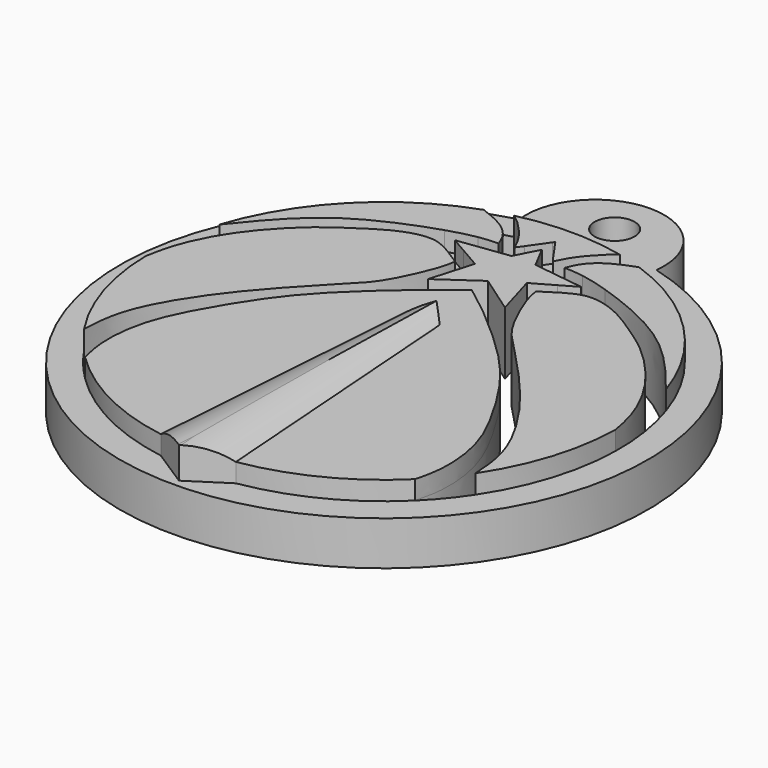
from build123d import *

# Parameters (mm, degrees)
F0_R        = 1.5875
F1_DEPTH    = 3.5
F2_DEPTH    = 5
F3_DEPTH    = 5
F4_DEPTH    = 6
F5_T1_DEPTH = 37.3647576307
F5_T3_DEPTH = 37.3647576307


# Not quite as in the source:
# - a fillet or chamfer that OpenCascade refuses, or shapes differently, is made with other operations: its cross-section is extruded or revolved along the edge and cut away or added


with BuildPart() as f1:
    # F0 (on Top) → F1 (new body)
    with BuildSketch(Plane.XY):
        with BuildLine():
            ThreePointArc((-10.6217474034, 18.1667311499), (-17.945936649, -18.7789449236), (15.8308902232, -2.1130307549))
            ThreePointArc((15.8308902232, -2.1130307549), (11.4968043919, 10.6637961173), (0.2835278497, 18.1667311499))
            ThreePointArc((0.2835278497, 18.1667311499), (-5.1691097768, 18.8869692451), (-10.6217474034, 18.1667311499))
        make_face()
        with BuildLine():
            ThreePointArc((7.9582883799, -15.4297572305), (3.287871388, -18.7906581631), (-2.183307789, -20.5724124585))
            Line((-2.183307789, -20.5724124585), (-5.1691097768, -22.5024949759))
            Line((-5.1691097768, -22.5024949759), (-8.1549117647, -20.5724124585))
            ThreePointArc((-8.1549117647, -20.5724124585), (-13.6260909417, -18.7906581631), (-18.2965079335, -15.4297572305))
            ThreePointArc((-18.2965079335, -15.4297572305), (-19.5901108284, -14.0167492942), (-20.7323538336, -12.4788023528))
            ThreePointArc((-20.7323538336, -12.4788023528), (-23.0163230381, -7.6934218882), (-23.8652020884, -2.4593235058))
            ThreePointArc((-23.8652020884, -2.4593235058), (-23.6597566898, 0.672604385), (-22.9333688875, 3.7260517623))
            ThreePointArc((-22.9333688875, 3.7260517623), (-18.5175516222, 10.9821166934), (-11.3474056156, 15.5361178626))
            ThreePointArc((-11.3474056156, 15.5361178626), (-10.3705266124, 15.8482901681), (-9.3780024098, 16.1064371078))
            ThreePointArc((-9.3780024098, 16.1064371078), (-5.1691097768, 16.5862683334), (-0.9602171439, 16.1064371078))
            ThreePointArc((-0.9602171439, 16.1064371078), (0.0323070587, 15.8482901681), (1.0091860619, 15.5361178626))
            ThreePointArc((1.0091860619, 15.5361178626), (8.1793320686, 10.9821166934), (12.5951493338, 3.7260517623))
            ThreePointArc((12.5951493338, 3.7260517623), (13.3215371361, 0.672604385), (13.5269825347, -2.4593235058))
            ThreePointArc((13.5269825347, -2.4593235058), (12.6781034844, -7.6934218882), (10.3941342799, -12.4788023528))
            ThreePointArc((10.3941342799, -12.4788023528), (9.2518912747, -14.0167492942), (7.9582883799, -15.4297572305))
        make_face(mode=Mode.SUBTRACT)
        with BuildLine():
            ThreePointArc((-10.6217474034, 18.1667311499), (-5.1691097768, 18.8869692451), (0.2835278497, 18.1667311499))
            ThreePointArc((0.2835278497, 18.1667311499), (-5.1691097768, 24.3869692451), (-10.6217474034, 18.1667311499))
        make_face()
        with Locations((-5.1691097768, 20.8305809647)):
            Circle(F0_R, mode=Mode.SUBTRACT)
        with BuildLine():
            Line((-3.8073558551, 1.7333009746), (-2.183307789, -20.5724124585))
            ThreePointArc((-2.183307789, -20.5724124585), (3.287871388, -18.7906581631), (7.9582883799, -15.4297572305))
            add(Edge.make_bspline(
                [(7.9582883799, -15.4297572305), (8.1268709506, -14.7676605332), (8.5082883638, -13.2407756078), (8.2126910715, -9.4168255285), (6.2922035042, -5.5331151551), (3.6366838506, -1.3148563239), (0.7165543738, 1.7563956632), (-2.917726549, 4.9627751379), (-4.4908734673, 6.1293824819), (-5.1691097768, 6.6323461942)],
                knots=[0, 0, 0, 0, 0.1082288162, 0.2489656613, 0.4027377179, 0.5651921966, 0.718242587, 0.878508978, 1, 1, 1, 1], degree=3))
            add(Edge.make_bspline(
                [(-18.2965079335, -15.4297572305), (-18.4650905043, -14.7676605332), (-18.8465079175, -13.2407756078), (-18.5509106252, -9.4168255285), (-16.6304230579, -5.5331151551), (-13.9749034043, -1.3148563239), (-11.0547739275, 1.7563956632), (-7.4204930047, 4.9627751379), (-5.8473460864, 6.1293824819), (-5.1691097768, 6.6323461942)],
                knots=[0, 0, 0, 0, 0.1082288162, 0.2489656613, 0.4027377179, 0.5651921966, 0.718242587, 0.878508978, 1, 1, 1, 1], degree=3))
            ThreePointArc((-18.2965079335, -15.4297572305), (-13.6260909417, -18.7906581631), (-8.1549117647, -20.5724124585))
            Line((-8.1549117647, -20.5724124585), (-6.5308636986, 1.7333009746))
            Line((-6.5308636986, 1.7333009746), (-5.1691097768, 3.1168696005))
            Line((-5.1691097768, 3.1168696005), (-3.8073558551, 1.7333009746))
        make_face()
    extrude(amount=F1_DEPTH)



with BuildPart() as f1b:
    # F0 (on Top) → F1, piece 2 (new body)
    with BuildSketch(Plane.XY):
        with BuildLine():
            add(Edge.make_bspline(
                [(-0.6594804695, 9.8146022568), (-0.3132768964, 10.0157483029), (0.352786766, 10.3622623091), (0.9138670644, 10.4710599705), (1.1655195088, 10.4825454153)],
                knots=[0.1007074481, 0.1007074481, 0.1007074481, 0.1007074481, 0.167295478, 0.2177868881, 0.2177868881, 0.2177868881, 0.2177868881], degree=3))
            ThreePointArc((1.1655195088, 10.4825454153), (1.3107635614, 10.8394988108), (1.3602674152, 11.2216779962))
            ThreePointArc((1.3602674152, 11.2216779962), (1.3218671337, 11.558911243), (1.2086323982, 11.878878021))
            add(Edge.make_bspline(
                [(1.2086323982, 11.878878021), (0.6116951762, 12.0699599932), (-0.1950310099, 12.2945209177), (-0.8204575004, 12.4165577745), (-1.0045308117, 12.4472896912)],
                knots=[0.7363290583, 0.7363290583, 0.7363290583, 0.7363290583, 0.8238242503, 0.864376936, 0.864376936, 0.864376936, 0.864376936], degree=3))
            ThreePointArc((-1.0045308117, 12.4472896912), (-1.4231996557, 11.9980234592), (-1.626745872, 11.4186335336))
            Line((-1.626745872, 11.4186335336), (-0.1397325848, 11.2216779962))
            Line((-0.1397325848, 11.2216779962), (-1.441368461, 10.4761955713))
            ThreePointArc((-1.441368461, 10.4761955713), (-1.1086423482, 10.076595523), (-0.6594804695, 9.8146022568))
        make_face()
    extrude(amount=F1_DEPTH)


with BuildPart() as f1c:
    # F0 (on Top) → F1, piece 3 (new body)
    with BuildSketch(Plane.XY):
        with BuildLine():
            ThreePointArc((-11.5468519519, 11.878878021), (-11.6977724933, 11.1753863528), (-11.5037390625, 10.4825454153))
            add(Edge.make_bspline(
                [(-9.6787390842, 9.8146022568), (-10.0249426572, 10.0157483029), (-10.6910063197, 10.3622623091), (-11.2520866181, 10.4710599705), (-11.5037390625, 10.4825454153)],
                knots=[0.1007074481, 0.1007074481, 0.1007074481, 0.1007074481, 0.167295478, 0.2177868881, 0.2177868881, 0.2177868881, 0.2177868881], degree=3))
            ThreePointArc((-9.6787390842, 9.8146022568), (-9.2295772055, 10.076595523), (-8.8968510927, 10.4761955713))
            Line((-8.8968510927, 10.4761955713), (-10.1984869689, 11.2216779962))
            Line((-10.1984869689, 11.2216779962), (-8.7114736817, 11.4186335336))
            ThreePointArc((-8.7114736817, 11.4186335336), (-8.915019898, 11.9980234592), (-9.333688742, 12.4472896912))
            add(Edge.make_bspline(
                [(-11.5468519519, 11.878878021), (-10.9499147299, 12.0699599932), (-10.1431885437, 12.2945209177), (-9.5177620533, 12.4165577745), (-9.333688742, 12.4472896912)],
                knots=[0.7363290583, 0.7363290583, 0.7363290583, 0.7363290583, 0.8238242503, 0.864376936, 0.864376936, 0.864376936, 0.864376936], degree=3))
        make_face()
    extrude(amount=F1_DEPTH)


with BuildPart() as f1d:
    # F0 (on Top) → F1, piece 4 (new body)
    with BuildSketch(Plane.XY):
        with BuildLine():
            ThreePointArc((-4.6168923991, 12.5363375369), (-4.2373473906, 12.8481972521), (-4.0154397933, 13.2864527868))
            add(Edge.make_bspline(
                [(-4.0154397933, 13.2864527868), (-4.1692049041, 13.4990699244), (-4.5365971578, 14.0110964025), (-4.8706595062, 14.4992054582), (-5.0654287777, 14.7850824568)],
                knots=[0.2267202191, 0.2267202191, 0.2267202191, 0.2267202191, 0.5150033084, 0.9268445188, 0.9268445188, 0.9268445188, 0.9268445188], degree=3))
            ThreePointArc((-5.0654287777, 14.7850824568), (-5.1691097768, 14.7895914288), (-5.272790776, 14.7850824568))
            add(Edge.make_bspline(
                [(-6.3227797603, 13.2864527868), (-6.1690146496, 13.4990699244), (-5.8016223959, 14.0110964025), (-5.4675600475, 14.4992054582), (-5.272790776, 14.7850824568)],
                knots=[0.2267202191, 0.2267202191, 0.2267202191, 0.2267202191, 0.5150033084, 0.9268445188, 0.9268445188, 0.9268445188, 0.9268445188], degree=3))
            ThreePointArc((-6.3227797603, 13.2864527868), (-6.1008721631, 12.8481972521), (-5.7213271546, 12.5363375369))
            Line((-5.7213271546, 12.5363375369), (-5.2771929481, 13.3880313451))
            Line((-5.2771929481, 13.3880313451), (-5.1691097768, 13.5952970013))
            Line((-5.1691097768, 13.5952970013), (-4.6168923991, 12.5363375369))
        make_face()
        with BuildLine():
            ThreePointArc((-5.7213271546, 12.5363375369), (-5.1691097768, 12.4010025738), (-4.6168923991, 12.5363375369))
            Line((-4.6168923991, 12.5363375369), (-5.1691097768, 13.5952970013))
            Line((-5.1691097768, 13.5952970013), (-5.2771929481, 13.3880313451))
            Line((-5.2771929481, 13.3880313451), (-5.7213271546, 12.5363375369))
        make_face()
    extrude(amount=F1_DEPTH)


with BuildPart() as f1_1:
    add(f1.part)

    add(f1b.part)  # F2 merges F1b

    add(f1c.part)  # F2 merges F1c

    add(f1d.part)  # F2 merges F1d
    # F0 (on Top) → F2 (join)
    with BuildSketch(Plane.XY):
        with BuildLine():
            Line((-3.8073558551, 1.7333009746), (-2.183307789, -20.5724124585))
            ThreePointArc((-2.183307789, -20.5724124585), (3.287871388, -18.7906581631), (7.9582883799, -15.4297572305))
            add(Edge.make_bspline(
                [(7.9582883799, -15.4297572305), (8.1268709506, -14.7676605332), (8.5082883638, -13.2407756078), (8.2126910715, -9.4168255285), (6.2922035042, -5.5331151551), (3.6366838506, -1.3148563239), (0.7165543738, 1.7563956632), (-2.917726549, 4.9627751379), (-4.4908734673, 6.1293824819), (-5.1691097768, 6.6323461942)],
                knots=[0, 0, 0, 0, 0.1082288162, 0.2489656613, 0.4027377179, 0.5651921966, 0.718242587, 0.878508978, 1, 1, 1, 1], degree=3))
            add(Edge.make_bspline(
                [(-18.2965079335, -15.4297572305), (-18.4650905043, -14.7676605332), (-18.8465079175, -13.2407756078), (-18.5509106252, -9.4168255285), (-16.6304230579, -5.5331151551), (-13.9749034043, -1.3148563239), (-11.0547739275, 1.7563956632), (-7.4204930047, 4.9627751379), (-5.8473460864, 6.1293824819), (-5.1691097768, 6.6323461942)],
                knots=[0, 0, 0, 0, 0.1082288162, 0.2489656613, 0.4027377179, 0.5651921966, 0.718242587, 0.878508978, 1, 1, 1, 1], degree=3))
            ThreePointArc((-18.2965079335, -15.4297572305), (-13.6260909417, -18.7906581631), (-8.1549117647, -20.5724124585))
            Line((-8.1549117647, -20.5724124585), (-6.5308636986, 1.7333009746))
            Line((-6.5308636986, 1.7333009746), (-5.1691097768, 3.1168696005))
            Line((-5.1691097768, 3.1168696005), (-3.8073558551, 1.7333009746))
        make_face()
        with BuildLine():
            add(Edge.make_bspline(
                [(10.3941342799, -12.4788023528), (10.3452942412, -11.6564178564), (10.2266128746, -9.932430264), (9.1917748323, -7.0399501633), (6.2457162099, -2.4988215533), (1.6434245686, 2.3032416473), (-0.1345824017, 4.0356531353), (-1.7597757021, 7.7058988796), (-1.8958501186, 8.6475784808), (-1.9455046584, 8.991218172)],
                knots=[0, 0, 0, 0, 0.1218601492, 0.2546294874, 0.4377987849, 0.6359398562, 0.762473885, 0.9132895155, 1, 1, 1, 1], degree=3))
            ThreePointArc((10.3941342799, -12.4788023528), (12.6781034844, -7.6934218882), (13.5269825347, -2.4593235058))
            add(Edge.make_bspline(
                [(1.1655195088, 10.4825454153), (1.3095245657, 10.4891178217), (1.9782324137, 10.4662598398), (3.6604034661, 10.0126361433), (6.3600557238, 8.1858017478), (8.468040147, 6.6827991764), (11.432590494, 3.4209544025), (13.0749001344, -0.038175844), (13.3944902979, -1.7190671567), (13.5269825347, -2.4593235058)],
                knots=[0.2177868881, 0.2177868881, 0.2177868881, 0.2177868881, 0.2466799847, 0.3490657461, 0.4784660181, 0.5963471121, 0.7469989964, 0.8886972052, 1, 1, 1, 1], degree=3))
            ThreePointArc((1.1655195088, 10.4825454153), (0.3758168612, 9.8130585413), (-0.6594804695, 9.8146022568))
            add(Edge.make_bspline(
                [(-1.9455046584, 8.991218172), (-1.6687696745, 9.1788138573), (-1.2974280921, 9.4305422257), (-0.7928309739, 9.737124932), (-0.6594804695, 9.8146022568)],
                knots=[0, 0, 0, 0, 0.075059107, 0.1007074481, 0.1007074481, 0.1007074481, 0.1007074481], degree=3))
        make_face()
        with BuildLine():
            add(Edge.make_bspline(
                [(12.5951493338, 3.7260517623), (11.837319685, 4.6792052854), (10.1727952981, 6.7348601777), (6.9410883324, 9.6905588931), (2.79917555, 11.3697388499), (1.2086323982, 11.878878021)],
                knots=[0, 0, 0, 0, 0.2320938274, 0.5031975443, 0.7363290583, 0.7363290583, 0.7363290583, 0.7363290583], degree=3))
            ThreePointArc((12.5951493338, 3.7260517623), (8.1793320686, 10.9821166934), (1.0091860619, 15.5361178626))
            add(Edge.make_bspline(
                [(-2.5381853063, 12.5784734264), (-2.4197419628, 12.891192737), (-2.1668564437, 13.5586539752), (-1.2444477594, 14.5311057124), (0.0078417422, 15.1550512291), (0.6915665814, 15.4186675749), (1.0091860619, 15.5361178626)],
                knots=[0, 0, 0, 0, 0.2315172069, 0.4938081985, 0.7644978013, 1, 1, 1, 1], degree=3))
            add(Edge.make_bspline(
                [(-1.0045308117, 12.4472896912), (-1.620139519, 12.5500684992), (-2.0791736657, 12.5642963988), (-2.5381853063, 12.5784734264)],
                knots=[0.864376936, 0.864376936, 0.864376936, 0.864376936, 1, 1, 1, 1], degree=3))
            ThreePointArc((-1.0045308117, 12.4472896912), (0.2334056719, 12.6745261787), (1.2086323982, 11.878878021))
        make_face()
        with BuildLine():
            ThreePointArc((-0.6594804695, 9.8146022568), (0.3758168612, 9.8130585413), (1.1655195088, 10.4825454153))
            add(Edge.make_bspline(
                [(-0.6594804695, 9.8146022568), (-0.3132768964, 10.0157483029), (0.352786766, 10.3622623091), (0.9138670644, 10.4710599705), (1.1655195088, 10.4825454153)],
                knots=[0.1007074481, 0.1007074481, 0.1007074481, 0.1007074481, 0.167295478, 0.2177868881, 0.2177868881, 0.2177868881, 0.2177868881], degree=3))
        make_face()
        with BuildLine():
            ThreePointArc((-23.8652020884, -2.4593235058), (-23.0163230381, -7.6934218882), (-20.7323538336, -12.4788023528))
            add(Edge.make_bspline(
                [(-20.7323538336, -12.4788023528), (-20.6835137949, -11.6564178564), (-20.5648324283, -9.932430264), (-19.529994386, -7.0399501633), (-16.5839357635, -2.4988215533), (-11.9816441223, 2.3032416473), (-10.2036371519, 4.0356531353), (-8.5784438516, 7.7058988796), (-8.4423694351, 8.6475784808), (-8.3927148953, 8.991218172)],
                knots=[0, 0, 0, 0, 0.1218601492, 0.2546294874, 0.4377987849, 0.6359398562, 0.762473885, 0.9132895155, 1, 1, 1, 1], degree=3))
            add(Edge.make_bspline(
                [(-8.3927148953, 8.991218172), (-8.6694498791, 9.1788138573), (-9.0407914616, 9.4305422257), (-9.5453885798, 9.737124932), (-9.6787390842, 9.8146022568)],
                knots=[0, 0, 0, 0, 0.075059107, 0.1007074481, 0.1007074481, 0.1007074481, 0.1007074481], degree=3))
            ThreePointArc((-9.6787390842, 9.8146022568), (-10.7140364149, 9.8130585413), (-11.5037390625, 10.4825454153))
            add(Edge.make_bspline(
                [(-11.5037390625, 10.4825454153), (-11.6477441193, 10.4891178217), (-12.3164519674, 10.4662598398), (-13.9986230197, 10.0126361433), (-16.6982752775, 8.1858017478), (-18.8062597007, 6.6827991764), (-21.7708100477, 3.4209544025), (-23.413119688, -0.038175844), (-23.7327098516, -1.7190671567), (-23.8652020884, -2.4593235058)],
                knots=[0.2177868881, 0.2177868881, 0.2177868881, 0.2177868881, 0.2466799847, 0.3490657461, 0.4784660181, 0.5963471121, 0.7469989964, 0.8886972052, 1, 1, 1, 1], degree=3))
        make_face()
        with BuildLine():
            add(Edge.make_bspline(
                [(1.2086323982, 11.878878021), (0.6116951762, 12.0699599932), (-0.1950310099, 12.2945209177), (-0.8204575004, 12.4165577745), (-1.0045308117, 12.4472896912)],
                knots=[0.7363290583, 0.7363290583, 0.7363290583, 0.7363290583, 0.8238242503, 0.864376936, 0.864376936, 0.864376936, 0.864376936], degree=3))
            ThreePointArc((1.2086323982, 11.878878021), (0.2334056719, 12.6745261787), (-1.0045308117, 12.4472896912))
        make_face()
        with BuildLine():
            add(Edge.make_bspline(
                [(-0.9602171439, 16.1064371078), (-1.1965800048, 15.9358141969), (-1.7643121989, 15.503844022), (-3.0700995974, 14.0384146087), (-3.4678370488, 13.175622067), (-3.6495767725, 12.7826062962)],
                knots=[0, 0, 0, 0, 0.2782728656, 0.6692240827, 1, 1, 1, 1], degree=3))
            ThreePointArc((-0.9602171439, 16.1064371078), (-5.1691097768, 16.5862683334), (-9.3780024098, 16.1064371078))
            add(Edge.make_bspline(
                [(-9.3780024098, 16.1064371078), (-9.1416395489, 15.9358141969), (-8.5739073548, 15.503844022), (-7.2681199563, 14.0384146087), (-6.8703825049, 13.175622067), (-6.6886427812, 12.7826062962)],
                knots=[0, 0, 0, 0, 0.2782728656, 0.6692240827, 1, 1, 1, 1], degree=3))
            add(Edge.make_bspline(
                [(-6.6886427812, 12.7826062962), (-6.5661755521, 12.9509231737), (-6.4437083229, 13.1192400511), (-6.3227797603, 13.2864527868)],
                knots=[0, 0, 0, 0, 0.2267202191, 0.2267202191, 0.2267202191, 0.2267202191], degree=3))
            ThreePointArc((-6.3227797603, 13.2864527868), (-6.1472230603, 14.2805951732), (-5.272790776, 14.7850824568))
            add(Edge.make_bspline(
                [(-5.272790776, 14.7850824568), (-5.2381938502, 14.8358628761), (-5.2036518135, 14.8866039073), (-5.1691097768, 14.9373449385)],
                knots=[0.9268445188, 0.9268445188, 0.9268445188, 0.9268445188, 1, 1, 1, 1], degree=3))
            add(Edge.make_bspline(
                [(-5.0654287777, 14.7850824568), (-5.1000257034, 14.8358628761), (-5.1345677401, 14.8866039073), (-5.1691097768, 14.9373449385)],
                knots=[0.9268445188, 0.9268445188, 0.9268445188, 0.9268445188, 1, 1, 1, 1], degree=3))
            ThreePointArc((-5.0654287777, 14.7850824568), (-4.2887221295, 14.4023018155), (-3.9748153493, 13.5952970013))
            ThreePointArc((-3.9748153493, 13.5952970013), (-3.9850150146, 13.4395447186), (-4.0154397933, 13.2864527868))
            add(Edge.make_bspline(
                [(-3.6495767725, 12.7826062962), (-3.7720440016, 12.9509231737), (-3.8945112308, 13.1192400511), (-4.0154397933, 13.2864527868)],
                knots=[0, 0, 0, 0, 0.2267202191, 0.2267202191, 0.2267202191, 0.2267202191], degree=3))
        make_face()
        with BuildLine():
            ThreePointArc((-11.3474056156, 15.5361178626), (-18.5175516222, 10.9821166934), (-22.9333688875, 3.7260517623))
            add(Edge.make_bspline(
                [(-22.9333688875, 3.7260517623), (-22.1755392387, 4.6792052854), (-20.5110148518, 6.7348601777), (-17.2793078861, 9.6905588931), (-13.1373951037, 11.3697388499), (-11.5468519519, 11.878878021)],
                knots=[0, 0, 0, 0, 0.2320938274, 0.5031975443, 0.7363290583, 0.7363290583, 0.7363290583, 0.7363290583], degree=3))
            ThreePointArc((-11.5468519519, 11.878878021), (-10.5716252256, 12.6745261787), (-9.333688742, 12.4472896912))
            add(Edge.make_bspline(
                [(-9.333688742, 12.4472896912), (-8.7180800347, 12.5500684992), (-8.2590458879, 12.5642963988), (-7.8000342473, 12.5784734264)],
                knots=[0.864376936, 0.864376936, 0.864376936, 0.864376936, 1, 1, 1, 1], degree=3))
            add(Edge.make_bspline(
                [(-7.8000342473, 12.5784734264), (-7.9184775909, 12.891192737), (-8.17136311, 13.5586539752), (-9.0937717943, 14.5311057124), (-10.3460612959, 15.1550512291), (-11.0297861351, 15.4186675749), (-11.3474056156, 15.5361178626)],
                knots=[0, 0, 0, 0, 0.2315172069, 0.4938081985, 0.7644978013, 1, 1, 1, 1], degree=3))
        make_face()
        with BuildLine():
            add(Edge.make_bspline(
                [(-9.6787390842, 9.8146022568), (-10.0249426572, 10.0157483029), (-10.6910063197, 10.3622623091), (-11.2520866181, 10.4710599705), (-11.5037390625, 10.4825454153)],
                knots=[0.1007074481, 0.1007074481, 0.1007074481, 0.1007074481, 0.167295478, 0.2177868881, 0.2177868881, 0.2177868881, 0.2177868881], degree=3))
            ThreePointArc((-11.5037390625, 10.4825454153), (-10.7140364149, 9.8130585413), (-9.6787390842, 9.8146022568))
        make_face()
        with BuildLine():
            ThreePointArc((-9.333688742, 12.4472896912), (-10.5716252256, 12.6745261787), (-11.5468519519, 11.878878021))
            add(Edge.make_bspline(
                [(-11.5468519519, 11.878878021), (-10.9499147299, 12.0699599932), (-10.1431885437, 12.2945209177), (-9.5177620533, 12.4165577745), (-9.333688742, 12.4472896912)],
                knots=[0.7363290583, 0.7363290583, 0.7363290583, 0.7363290583, 0.8238242503, 0.864376936, 0.864376936, 0.864376936, 0.864376936], degree=3))
        make_face()
        with BuildLine():
            add(Edge.make_bspline(
                [(-4.0154397933, 13.2864527868), (-4.1692049041, 13.4990699244), (-4.5365971578, 14.0110964025), (-4.8706595062, 14.4992054582), (-5.0654287777, 14.7850824568)],
                knots=[0.2267202191, 0.2267202191, 0.2267202191, 0.2267202191, 0.5150033084, 0.9268445188, 0.9268445188, 0.9268445188, 0.9268445188], degree=3))
            ThreePointArc((-4.0154397933, 13.2864527868), (-3.9850150146, 13.4395447186), (-3.9748153493, 13.5952970013))
            ThreePointArc((-3.9748153493, 13.5952970013), (-4.2887221295, 14.4023018155), (-5.0654287777, 14.7850824568))
        make_face()
        with BuildLine():
            ThreePointArc((-5.7213271546, 12.5363375369), (-5.1691097768, 12.4010025738), (-4.6168923991, 12.5363375369))
            Line((-4.6168923991, 12.5363375369), (-5.1691097768, 13.5952970013))
            Line((-5.1691097768, 13.5952970013), (-5.2771929481, 13.3880313451))
            Line((-5.2771929481, 13.3880313451), (-5.7213271546, 12.5363375369))
        make_face()
        with BuildLine():
            ThreePointArc((-5.272790776, 14.7850824568), (-6.1472230603, 14.2805951732), (-6.3227797603, 13.2864527868))
            add(Edge.make_bspline(
                [(-6.3227797603, 13.2864527868), (-6.1690146496, 13.4990699244), (-5.8016223959, 14.0110964025), (-5.4675600475, 14.4992054582), (-5.272790776, 14.7850824568)],
                knots=[0.2267202191, 0.2267202191, 0.2267202191, 0.2267202191, 0.5150033084, 0.9268445188, 0.9268445188, 0.9268445188, 0.9268445188], degree=3))
        make_face()
    extrude(amount=F2_DEPTH)

    # F0 (on Top) → F3 (join)
    with BuildSketch(Plane.XY):
        Polygon((-5.1691097768, -22.5024949759), (-2.183307789, -20.5724124585), (-3.8073558551, 1.7333009746), (-5.1691097768, 3.1168696005), (-6.5308636986, 1.7333009746), (-8.1549117647, -20.5724124585), align=None)
        with BuildLine():
            ThreePointArc((-1.626745872, 11.4186335336), (-1.61153025, 10.9321756081), (-1.441368461, 10.4761955713))
            Line((-1.441368461, 10.4761955713), (-0.1397325848, 11.2216779962))
            Line((-0.1397325848, 11.2216779962), (-1.626745872, 11.4186335336))
        make_face()
        with BuildLine():
            Line((-3.1067568068, 9.52238217), (-1.441368461, 10.4761955713))
            ThreePointArc((-1.441368461, 10.4761955713), (-1.61153025, 10.9321756081), (-1.626745872, 11.4186335336))
            Line((-1.626745872, 11.4186335336), (-4.2126474162, 11.7611372843))
            Line((-4.2126474162, 11.7611372843), (-4.6168923991, 12.5363375369))
            ThreePointArc((-4.6168923991, 12.5363375369), (-5.1691097768, 12.4010025738), (-5.7213271546, 12.5363375369))
            Line((-5.7213271546, 12.5363375369), (-6.1255721375, 11.7611372843))
            Line((-6.1255721375, 11.7611372843), (-8.7114736817, 11.4186335336))
            ThreePointArc((-8.7114736817, 11.4186335336), (-8.7017371683, 11.3203696099), (-8.6984869689, 11.2216779962))
            ThreePointArc((-8.6984869689, 11.2216779962), (-8.7489260329, 10.8359668441), (-8.8968510927, 10.4761955713))
            Line((-8.8968510927, 10.4761955713), (-7.2314627469, 9.52238217))
            Line((-7.2314627469, 9.52238217), (-8.2294614986, 6.0968184844))
            Line((-8.2294614986, 6.0968184844), (-5.1691097768, 8.2276808098))
            Line((-5.1691097768, 8.2276808098), (-2.1087580551, 6.0968184844))
            Line((-2.1087580551, 6.0968184844), (-3.1067568068, 9.52238217))
        make_face()
        with BuildLine():
            Line((-10.1984869689, 11.2216779962), (-8.8968510927, 10.4761955713))
            ThreePointArc((-8.8968510927, 10.4761955713), (-8.7489260329, 10.8359668441), (-8.6984869689, 11.2216779962))
            ThreePointArc((-8.6984869689, 11.2216779962), (-8.7017371683, 11.3203696099), (-8.7114736817, 11.4186335336))
            Line((-8.7114736817, 11.4186335336), (-10.1984869689, 11.2216779962))
        make_face()
    extrude(amount=F3_DEPTH)

    # F0 (on Top) → F4 (join)
    with BuildSketch(Plane.XY):
        Polygon((-5.1691097768, -22.5024949759), (-2.183307789, -20.5724124585), (-3.8073558551, 1.7333009746), (-5.1691097768, 3.1168696005), (-6.5308636986, 1.7333009746), (-8.1549117647, -20.5724124585), align=None)
    extrude(amount=F4_DEPTH)

    # F5: fillet of radius 5 on 2 edges, made by hand

    # F5_s2 → F5_t1 (cut)
    with BuildSketch(Plane(origin=(0.6357185704, 8.7313648843, 0), x_dir=(0, 0, 1), z_dir=(-0.0726163946, -0.9973599447, 0))):
        with BuildLine():
            ThreePointArc((5, 6.6394879246), (5.7434164903, 5.2206267547), (6, 3.6394879246))
            Line((6, 3.6394879246), (6, 6.6394879246))
            Line((6, 6.6394879246), (5, 6.6394879246))
        make_face()
    extrude(amount=F5_T1_DEPTH, mode=Mode.SUBTRACT)

    # F5_s4 → F5_t3 (cut)
    with BuildSketch(Plane(origin=(2.0230605283, -27.7860054414, 0), x_dir=(0, 0, 1), z_dir=(-0.0726163946, 0.9973599447, 0))):
        with BuildLine():
            ThreePointArc((5, -3.6714381574), (5.7434164903, -5.0902993273), (6, -6.6714381574))
            Line((6, -6.6714381574), (6, -3.6714381574))
            Line((6, -3.6714381574), (5, -3.6714381574))
        make_face()
    extrude(amount=F5_T3_DEPTH, mode=Mode.SUBTRACT)


solid = f1_1.part
